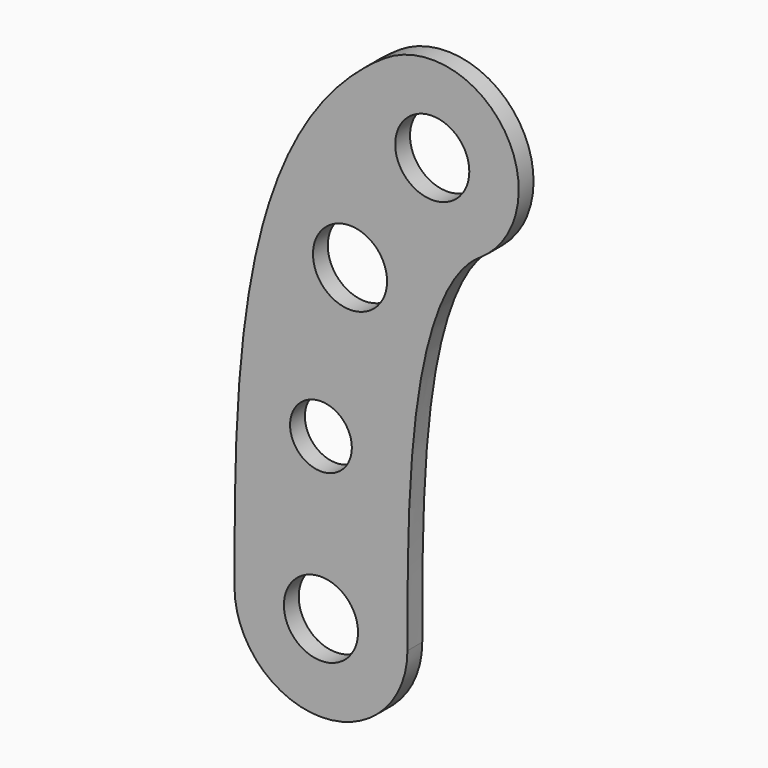
from build123d import *

# Parameters (mm, degrees)
F0_R     = 6
F1_DEPTH = 3
F3_R     = 5
F4_DEPTH = 9.4
F5_R     = 5
F6_DEPTH = 2


# Not quite as in the source:
# - ends of sketch curves that miss each other by under 0.0002 mm in the source are joined
# - the dataset's text gives a spline's control points without its knots; the knots are read off the source's solid


with BuildPart() as f1:
    # F0 (on Front) → F1 (new body)
    with BuildSketch(Plane.XZ):
        with BuildLine():
            add(Edge.make_bspline(
                [(-14, -26), (-14, -22.75), (-14.0004523743, -15.9105291262), (-13.7828666825, -5.0097493319), (-13.1111411806, 6.2097947293), (-11.720563989, 17.4707102353), (-9.6943656003, 26.7000282147), (-7.3231272908, 33.8894297819), (-5.0899646489, 39.15233442), (-2.3107556278, 44.2379137207), (1.1152604329, 49.0651401417), (5.2757801793, 53.5029660938), (8.5623848122, 56.0788774956), (10.3247279458, 57.2378033443)],
                knots=[0, 0, 0, 0, 0.125, 0.25, 0.375, 0.5, 0.625, 0.6875, 0.75, 0.8125, 0.875, 0.9375, 1, 1, 1, 1], degree=3))
            ThreePointArc((-14, -26), (0, -40), (14, -26))
            add(Edge.make_bspline(
                [(14, -26), (14, -22.75), (14.0004523743, -16.1086995406), (14.205139987, -6.0382727532), (14.8002343988, 3.7711749321), (15.9432970346, 12.9047719201), (17.4360428506, 19.5652612944), (18.9356431663, 24.0782015665), (20.186235287, 27.0007682339), (21.5241909854, 29.4228421126), (22.9015337641, 31.3389176928), (24.2833500376, 32.7935083509), (25.2194773121, 33.5209300274), (25.7092571932, 33.8430120472)],
                knots=[0, 0, 0, 0, 0.125, 0.25, 0.375, 0.5, 0.625, 0.6875, 0.75, 0.8125, 0.875, 0.9375, 0.9999998504, 0.9999998504, 0.9999998504, 0.9999998504], degree=3))
            ThreePointArc((25.7092571932, 33.8430120472), (29.7143803557, 53.2326803132), (10.3247279458, 57.2378033443))
        make_face()
        with Locations((0, -26)):
            Circle(F0_R, mode=Mode.SUBTRACT)
        with Locations((4.704827633, 25.5707762288)):
            Circle(F0_R, mode=Mode.SUBTRACT)
        with Locations((18.0169899591, 45.5404115335)):
            Circle(F0_R, mode=Mode.SUBTRACT)
    extrude(amount=F1_DEPTH)


with BuildPart() as f2_1:
    # F2: copy of F1
    add(f1.part.moved(Location((50.8967, 0, 0))))

    # F3 (on face) → F4 (cut)
    with BuildSketch(Plane.XZ.offset(3)):
        with Locations((50.8965918246, 0)):
            Circle(F3_R)
    extrude(amount=-F4_DEPTH, mode=Mode.SUBTRACT)


with BuildPart() as f1_1:
    add(f1.part)

    # F5 (on face) → F6 (cut)
    with BuildSketch(Plane(origin=(0, 0, 0), x_dir=(-1, 0, 0), z_dir=(0, 1, 0))):
        Circle(F5_R)
    extrude(amount=-F6_DEPTH, mode=Mode.SUBTRACT)


solid = f2_1.part
